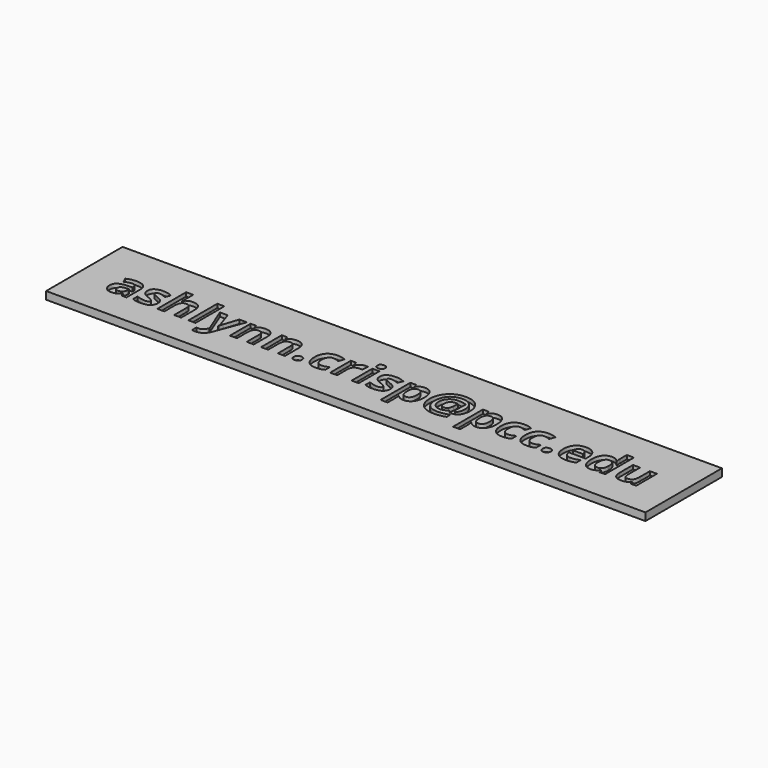
from build123d import *

# Parameters (mm, degrees)
F0_W         = 78
F0_H         = 12.4420574262
F0_W_2       = 0.9186807134
F0_H_2       = 3.3681746196
F0_H_3       = 4.6878744061
F0_TEXT_SIZE = 6.169524203
F1_DEPTH     = 1
F2_DEPTH     = 0.5


# Not quite as in the source:
# - Text() gives the source's letters only with a copy of the font that has no kerning and outlines rounded to 1/6400 em; it was checked with that copy


with BuildPart() as f1:
    # F0 (on Top) → F1 (new body)
    with BuildSketch(Plane.XY):
        with Locations((0, 2.2210287131)):
            Rectangle(F0_W, F0_H)
        with BuildLine():
            Line((-31.7378640777, 0), (-32.3789162019, 0))
            Line((-32.3789162019, 0), (-32.5572540109, 0.4578943744))
            Line((-32.5572540109, 0.4578943744), (-32.5813537148, 0.4578943744))
            add(Edge.make_bspline(
                [(-32.5813537148, 0.4578943744), (-32.8127108724, 0.165805963), (-33.0585278524, 0.0525373545)],
                knots=[0, 0, 0, 1, 1, 1], degree=2))
            add(Edge.make_bspline(
                [(-33.0585278524, 0.0525373545), (-33.3043448323, -0.0607312539), (-33.6986159884, -0.0607312539)],
                knots=[0, 0, 0, 1, 1, 1], degree=2))
            add(Edge.make_bspline(
                [(-33.6986159884, -0.0607312539), (-34.1835020313, -0.0607312539), (-34.4620946086, 0.2168973353)],
                knots=[0, 0, 0, 1, 1, 1], degree=2))
            add(Edge.make_bspline(
                [(-34.4620946086, 0.2168973353), (-34.7406871858, 0.4945259244), (-34.7406871858, 1.0064036356)],
                knots=[0, 0, 0, 1, 1, 1], degree=2))
            add(Edge.make_bspline(
                [(-34.7406871858, 1.0064036356), (-34.7406871858, 1.5423810507), (-34.3656957929, 1.7968739241)],
                knots=[0, 0, 0, 1, 1, 1], degree=2))
            add(Edge.make_bspline(
                [(-34.3656957929, 1.7968739241), (-33.9907043999, 2.0513667975), (-33.2349376851, 2.0783584659)],
                knots=[0, 0, 0, 1, 1, 1], degree=2))
            Line((-33.2349376851, 2.0783584659), (-32.6497968739, 2.0966742409))
            Line((-32.6497968739, 2.0966742409), (-32.6497968739, 2.2441644288))
            add(Edge.make_bspline(
                [(-32.6497968739, 2.2441644288), (-32.6497968739, 2.7560421401), (-33.1742064312, 2.7560421401)],
                knots=[0, 0, 0, 1, 1, 1], degree=2))
            add(Edge.make_bspline(
                [(-33.1742064312, 2.7560421401), (-33.5781174688, 2.7560421401), (-34.1237347655, 2.5121531364)],
                knots=[0, 0, 0, 1, 1, 1], degree=2))
            Line((-34.1237347655, 2.5121531364), (-34.4273910349, 3.1329615093))
            add(Edge.make_bspline(
                [(-34.4273910349, 3.1329615093), (-33.8461061764, 3.4375817669), (-33.1385388694, 3.4375817669)],
                knots=[0, 0, 0, 1, 1, 1], degree=2))
            add(Edge.make_bspline(
                [(-33.1385388694, 3.4375817669), (-32.4608551952, 3.4375817669), (-32.0993596364, 3.1421193968)],
                knots=[0, 0, 0, 1, 1, 1], degree=2))
            add(Edge.make_bspline(
                [(-32.0993596364, 3.1421193968), (-31.7378640777, 2.8466570268), (-31.7378640777, 2.2441644288)],
                knots=[0, 0, 0, 1, 1, 1], degree=2))
            Line((-31.7378640777, 2.2441644288), (-31.7378640777, 0))
        make_face(mode=Mode.SUBTRACT)
        with BuildLine():
            add(Edge.make_bspline(
                [(-28.528747504, 1.4310404186), (-28.4410245817, 1.2502926393), (-28.4410245817, 1.0006197067)],
                knots=[0, 0, 0, 1, 1, 1], degree=2))
            add(Edge.make_bspline(
                [(-28.4410245817, 1.0006197067), (-28.4410245817, 0.4819940784), (-28.8010741582, 0.2106314122)],
                knots=[0, 0, 0, 1, 1, 1], degree=2))
            add(Edge.make_bspline(
                [(-28.8010741582, 0.2106314122), (-29.1611237348, -0.0607312539), (-29.8783309234, -0.0607312539)],
                knots=[0, 0, 0, 1, 1, 1], degree=2))
            add(Edge.make_bspline(
                [(-29.8783309234, -0.0607312539), (-30.2456104111, -0.0607312539), (-30.5049232252, -0.0106038697)],
                knots=[0, 0, 0, 1, 1, 1], degree=2))
            add(Edge.make_bspline(
                [(-30.5049232252, -0.0106038697), (-30.7642360394, 0.0395235144), (-30.9898092681, 0.1359223301)],
                knots=[0, 0, 0, 1, 1, 1], degree=2))
            Line((-30.9898092681, 0.1359223301), (-30.9898092681, 0.8945810094))
            add(Edge.make_bspline(
                [(-30.9898092681, 0.8945810094), (-30.7343524065, 0.7740824898), (-30.4133443503, 0.6926254906)],
                knots=[0, 0, 0, 1, 1, 1], degree=2))
            add(Edge.make_bspline(
                [(-30.4133443503, 0.6926254906), (-30.0923362942, 0.6111684914), (-29.8484472905, 0.6111684914)],
                knots=[0, 0, 0, 1, 1, 1], degree=2))
            add(Edge.make_bspline(
                [(-29.8484472905, 0.6111684914), (-29.3481374372, 0.6111684914), (-29.3481374372, 0.9003649384)],
                knots=[0, 0, 0, 1, 1, 1], degree=2))
            add(Edge.make_bspline(
                [(-29.3481374372, 0.9003649384), (-29.3481374372, 1.0092956001), (-29.41465262, 1.0772567651)],
                knots=[0, 0, 0, 1, 1, 1], degree=2))
            add(Edge.make_bspline(
                [(-29.41465262, 1.0772567651), (-29.4811678028, 1.1452179302), (-29.6435998072, 1.2310128761)],
                knots=[0, 0, 0, 1, 1, 1], degree=2))
            add(Edge.make_bspline(
                [(-29.6435998072, 1.2310128761), (-29.8060318116, 1.3168078221), (-30.0769124836, 1.4305584246)],
                knots=[0, 0, 0, 1, 1, 1], degree=2))
            add(Edge.make_bspline(
                [(-30.0769124836, 1.4305584246), (-30.4653997108, 1.5934724231), (-30.6480754665, 1.7322867176)],
                knots=[0, 0, 0, 1, 1, 1], degree=2))
            add(Edge.make_bspline(
                [(-30.6480754665, 1.7322867176), (-30.8307512222, 1.8711010122), (-30.9131722096, 2.0504028093)],
                knots=[0, 0, 0, 1, 1, 1], degree=2))
            add(Edge.make_bspline(
                [(-30.9131722096, 2.0504028093), (-30.995593197, 2.2297046065), (-30.995593197, 2.490945397)],
                knots=[0, 0, 0, 1, 1, 1], degree=2))
            add(Edge.make_bspline(
                [(-30.995593197, 2.490945397), (-30.995593197, 2.940163878), (-30.6480754665, 3.1854988639)],
                knots=[0, 0, 0, 1, 1, 1], degree=2))
            add(Edge.make_bspline(
                [(-30.6480754665, 3.1854988639), (-30.300557736, 3.4308338498), (-29.6614335881, 3.4308338498)],
                knots=[0, 0, 0, 1, 1, 1], degree=2))
            add(Edge.make_bspline(
                [(-29.6614335881, 3.4308338498), (-29.0531570612, 3.4308338498), (-28.4776561317, 3.1657371067)],
                knots=[0, 0, 0, 1, 1, 1], degree=2))
            Line((-28.4776561317, 3.1657371067), (-28.7543207326, 2.503477243))
            add(Edge.make_bspline(
                [(-28.7543207326, 2.503477243), (-29.0078496178, 2.6114439165), (-29.2276389176, 2.6808510638)],
                knots=[0, 0, 0, 1, 1, 1], degree=2))
            add(Edge.make_bspline(
                [(-29.2276389176, 2.6808510638), (-29.4474282173, 2.7502582111), (-29.6768573986, 2.7502582111)],
                knots=[0, 0, 0, 1, 1, 1], degree=2))
            add(Edge.make_bspline(
                [(-29.6768573986, 2.7502582111), (-30.0836604007, 2.7502582111), (-30.0836604007, 2.5304689114)],
                knots=[0, 0, 0, 1, 1, 1], degree=2))
            add(Edge.make_bspline(
                [(-30.0836604007, 2.5304689114), (-30.0836604007, 2.4070784273), (-29.9525580114, 2.3164635406)],
                knots=[0, 0, 0, 1, 1, 1], degree=2))
            add(Edge.make_bspline(
                [(-29.9525580114, 2.3164635406), (-29.8214556221, 2.2258486539), (-29.37802107, 2.048474833)],
                knots=[0, 0, 0, 1, 1, 1], degree=2))
            add(Edge.make_bspline(
                [(-29.37802107, 2.048474833), (-28.9837499139, 1.888452799), (-28.8001101701, 1.7501204985)],
                knots=[0, 0, 0, 1, 1, 1], degree=2))
            add(Edge.make_bspline(
                [(-28.8001101701, 1.7501204985), (-28.6164704262, 1.611788198), (-28.528747504, 1.4310404186)],
                knots=[0, 0, 0, 1, 1, 1], degree=2))
        make_face(mode=Mode.SUBTRACT)
        with BuildLine():
            Line((-20.9315568409, 0.0240997039), (-22.2695724024, 3.3681746196))
            Line((-22.2695724024, 3.3681746196), (-21.2631687668, 3.3681746196))
            Line((-21.2631687668, 3.3681746196), (-20.6279005715, 1.4729739035))
            add(Edge.make_bspline(
                [(-20.6279005715, 1.4729739035), (-20.5459615782, 1.2261929353), (-20.5160779453, 0.8887970805)],
                knots=[0, 0, 0, 1, 1, 1], degree=2))
            Line((-20.5160779453, 0.8887970805), (-20.4977621704, 0.8887970805))
            add(Edge.make_bspline(
                [(-20.4977621704, 0.8887970805), (-20.464986573, 1.199201267), (-20.3685877574, 1.4729739035)],
                knots=[0, 0, 0, 1, 1, 1], degree=2))
            Line((-20.3685877574, 1.4729739035), (-19.74488742, 3.3681746196))
            Line((-19.74488742, 3.3681746196), (-18.7596915238, 3.3681746196))
            Line((-18.7596915238, 3.3681746196), (-20.1844660194, -0.4309027061))
            add(Edge.make_bspline(
                [(-20.1844660194, -0.4309027061), (-20.3811196034, -0.9582042278), (-20.7440611444, -1.2204090064)],
                knots=[0, 0, 0, 1, 1, 1], degree=2))
            add(Edge.make_bspline(
                [(-20.7440611444, -1.2204090064), (-21.1070026854, -1.482613785), (-21.5918887282, -1.482613785)],
                knots=[0, 0, 0, 1, 1, 1], degree=2))
            add(Edge.make_bspline(
                [(-21.5918887282, -1.482613785), (-21.8299938029, -1.482613785), (-22.0584589961, -1.4305584246)],
                knots=[0, 0, 0, 1, 1, 1], degree=2))
            Line((-22.0584589961, -1.4305584246), (-22.0584589961, -0.7017833781))
            add(Edge.make_bspline(
                [(-22.0584589961, -0.7017833781), (-21.8926530331, -0.7413068925), (-21.6969634373, -0.7413068925)],
                knots=[0, 0, 0, 1, 1, 1], degree=2))
            add(Edge.make_bspline(
                [(-21.6969634373, -0.7413068925), (-21.4530744337, -0.7413068925), (-21.270880672, -0.5918887282)],
                knots=[0, 0, 0, 1, 1, 1], degree=2))
            add(Edge.make_bspline(
                [(-21.270880672, -0.5918887282), (-21.0886869104, -0.4424705639), (-20.9865041658, -0.141706259)],
                knots=[0, 0, 0, 1, 1, 1], degree=2))
            Line((-20.9865041658, -0.141706259), (-20.9315568409, 0.0240997039))
        make_face(mode=Mode.SUBTRACT)
        with BuildLine():
            add(Edge.make_bspline(
                [(-10.1594711836, 0.0530193486), (-10.2978034841, 0.1870137024), (-10.2978034841, 0.4309027061)],
                knots=[0, 0, 0, 1, 1, 1], degree=2))
            add(Edge.make_bspline(
                [(-10.2978034841, 0.4309027061), (-10.2978034841, 0.6834676031), (-10.1623631481, 0.8131240102)],
                knots=[0, 0, 0, 1, 1, 1], degree=2))
            add(Edge.make_bspline(
                [(-10.1623631481, 0.8131240102), (-10.0269228121, 0.9427804173), (-9.7676099979, 0.9427804173)],
                knots=[0, 0, 0, 1, 1, 1], degree=2))
            add(Edge.make_bspline(
                [(-9.7676099979, 0.9427804173), (-9.5179370653, 0.9427804173), (-9.3810507471, 0.8102320457)],
                knots=[0, 0, 0, 1, 1, 1], degree=2))
            add(Edge.make_bspline(
                [(-9.3810507471, 0.8102320457), (-9.2441644288, 0.6776836742), (-9.2441644288, 0.4309027061)],
                knots=[0, 0, 0, 1, 1, 1], degree=2))
            add(Edge.make_bspline(
                [(-9.2441644288, 0.4309027061), (-9.2441644288, 0.1927976313), (-9.3824967293, 0.0559113131)],
                knots=[0, 0, 0, 1, 1, 1], degree=2))
            add(Edge.make_bspline(
                [(-9.3824967293, 0.0559113131), (-9.5208290298, -0.0809750052), (-9.7676099979, -0.0809750052)],
                knots=[0, 0, 0, 1, 1, 1], degree=2))
            add(Edge.make_bspline(
                [(-9.7676099979, -0.0809750052), (-10.0211388832, -0.0809750052), (-10.1594711836, 0.0530193486)],
                knots=[0, 0, 0, 1, 1, 1], degree=2))
        make_face(mode=Mode.SUBTRACT)
        with BuildLine():
            Line((-15.16883564, 2.195965021), (-15.16883564, 0))
            Line((-15.16883564, 0), (-16.0875163534, 0))
            Line((-16.0875163534, 0), (-16.0875163534, 1.9674998279))
            add(Edge.make_bspline(
                [(-16.0875163534, 1.9674998279), (-16.0875163534, 2.3318873511), (-16.2171727604, 2.5140811127)],
                knots=[0, 0, 0, 1, 1, 1], degree=2))
            add(Edge.make_bspline(
                [(-16.2171727604, 2.5140811127), (-16.3468291675, 2.6962748743), (-16.6302416856, 2.6962748743)],
                knots=[0, 0, 0, 1, 1, 1], degree=2))
            add(Edge.make_bspline(
                [(-16.6302416856, 2.6962748743), (-17.0158369483, 2.6962748743), (-17.1874268402, 2.4388900365)],
                knots=[0, 0, 0, 1, 1, 1], degree=2))
            add(Edge.make_bspline(
                [(-17.1874268402, 2.4388900365), (-17.3590167321, 2.1815051987), (-17.3590167321, 1.5847965296)],
                knots=[0, 0, 0, 1, 1, 1], degree=2))
            Line((-17.3590167321, 1.5847965296), (-17.3590167321, 0))
            Line((-17.3590167321, 0), (-18.2776974454, 0))
            Line((-18.2776974454, 0), (-18.2776974454, 3.3681746196))
            Line((-18.2776974454, 3.3681746196), (-17.5759140673, 3.3681746196))
            Line((-17.5759140673, 3.3681746196), (-17.4525235833, 2.9372719135))
            Line((-17.4525235833, 2.9372719135), (-17.401432211, 2.9372719135))
            add(Edge.make_bspline(
                [(-17.401432211, 2.9372719135), (-17.2471941059, 3.1811609172), (-16.9777594161, 3.3059973835)],
                knots=[0, 0, 0, 1, 1, 1], degree=2))
            add(Edge.make_bspline(
                [(-16.9777594161, 3.3059973835), (-16.7083247263, 3.4308338498), (-16.3651449425, 3.4308338498)],
                knots=[0, 0, 0, 1, 1, 1], degree=2))
            add(Edge.make_bspline(
                [(-16.3651449425, 3.4308338498), (-15.7771121669, 3.4308338498), (-15.4729739035, 3.1131997521)],
                knots=[0, 0, 0, 1, 1, 1], degree=2))
            add(Edge.make_bspline(
                [(-15.4729739035, 3.1131997521), (-15.16883564, 2.7955656545), (-15.16883564, 2.195965021)],
                knots=[0, 0, 0, 1, 1, 1], degree=2))
        make_face(mode=Mode.SUBTRACT)
        with BuildLine():
            Line((-11.1143014529, 2.195965021), (-11.1143014529, 0))
            Line((-11.1143014529, 0), (-12.0329821662, 0))
            Line((-12.0329821662, 0), (-12.0329821662, 1.9674998279))
            add(Edge.make_bspline(
                [(-12.0329821662, 1.9674998279), (-12.0329821662, 2.3318873511), (-12.1626385733, 2.5140811127)],
                knots=[0, 0, 0, 1, 1, 1], degree=2))
            add(Edge.make_bspline(
                [(-12.1626385733, 2.5140811127), (-12.2922949804, 2.6962748743), (-12.5757074985, 2.6962748743)],
                knots=[0, 0, 0, 1, 1, 1], degree=2))
            add(Edge.make_bspline(
                [(-12.5757074985, 2.6962748743), (-12.9613027611, 2.6962748743), (-13.132892653, 2.4388900365)],
                knots=[0, 0, 0, 1, 1, 1], degree=2))
            add(Edge.make_bspline(
                [(-13.132892653, 2.4388900365), (-13.3044825449, 2.1815051987), (-13.3044825449, 1.5847965296)],
                knots=[0, 0, 0, 1, 1, 1], degree=2))
            Line((-13.3044825449, 1.5847965296), (-13.3044825449, 0))
            Line((-13.3044825449, 0), (-14.2231632583, 0))
            Line((-14.2231632583, 0), (-14.2231632583, 3.3681746196))
            Line((-14.2231632583, 3.3681746196), (-13.5213798802, 3.3681746196))
            Line((-13.5213798802, 3.3681746196), (-13.3979893961, 2.9372719135))
            Line((-13.3979893961, 2.9372719135), (-13.3468980238, 2.9372719135))
            add(Edge.make_bspline(
                [(-13.3468980238, 2.9372719135), (-13.1926599187, 3.1811609172), (-12.9232252289, 3.3059973835)],
                knots=[0, 0, 0, 1, 1, 1], degree=2))
            add(Edge.make_bspline(
                [(-12.9232252289, 3.3059973835), (-12.6537905391, 3.4308338498), (-12.3106107554, 3.4308338498)],
                knots=[0, 0, 0, 1, 1, 1], degree=2))
            add(Edge.make_bspline(
                [(-12.3106107554, 3.4308338498), (-11.7225779798, 3.4308338498), (-11.4184397163, 3.1131997521)],
                knots=[0, 0, 0, 1, 1, 1], degree=2))
            add(Edge.make_bspline(
                [(-11.4184397163, 3.1131997521), (-11.1143014529, 2.7955656545), (-11.1143014529, 2.195965021)],
                knots=[0, 0, 0, 1, 1, 1], degree=2))
        make_face(mode=Mode.SUBTRACT)
        with BuildLine():
            add(Edge.make_bspline(
                [(-6.4678785375, -0.006265923), (-6.6953797425, -0.0607312539), (-7.0414514907, -0.0607312539)],
                knots=[0, 0, 0, 1, 1, 1], degree=2))
            add(Edge.make_bspline(
                [(-7.0414514907, -0.0607312539), (-8.6137161743, -0.0607312539), (-8.6137161743, 1.6657715348)],
                knots=[0, 0, 0, 1, 1, 1], degree=2))
            add(Edge.make_bspline(
                [(-8.6137161743, 1.6657715348), (-8.6137161743, 2.5246849824), (-8.1861874268, 2.9777594161)],
                knots=[0, 0, 0, 1, 1, 1], degree=2))
            add(Edge.make_bspline(
                [(-8.1861874268, 2.9777594161), (-7.7586586793, 3.4308338498), (-6.9604764856, 3.4308338498)],
                knots=[0, 0, 0, 1, 1, 1], degree=2))
            add(Edge.make_bspline(
                [(-6.9604764856, 3.4308338498), (-6.3762996626, 3.4308338498), (-5.9116573711, 3.2023686566)],
                knots=[0, 0, 0, 1, 1, 1], degree=2))
            Line((-5.9116573711, 3.2023686566), (-6.1835020313, 2.490945397))
            add(Edge.make_bspline(
                [(-6.1835020313, 2.490945397), (-6.4003993665, 2.5786683192), (-6.5869310748, 2.6345796323)],
                knots=[0, 0, 0, 1, 1, 1], degree=2))
            add(Edge.make_bspline(
                [(-6.5869310748, 2.6345796323), (-6.7734627832, 2.6904909454), (-6.9604764856, 2.6904909454)],
                knots=[0, 0, 0, 1, 1, 1], degree=2))
            add(Edge.make_bspline(
                [(-6.9604764856, 2.6904909454), (-7.6776836742, 2.6904909454), (-7.6776836742, 1.6715554637)],
                knots=[0, 0, 0, 1, 1, 1], degree=2))
            add(Edge.make_bspline(
                [(-7.6776836742, 1.6715554637), (-7.6776836742, 0.6834676031), (-6.9604764856, 0.6834676031)],
                knots=[0, 0, 0, 1, 1, 1], degree=2))
            add(Edge.make_bspline(
                [(-6.9604764856, 0.6834676031), (-6.6953797425, 0.6834676031), (-6.4693245197, 0.7543207326)],
                knots=[0, 0, 0, 1, 1, 1], degree=2))
            add(Edge.make_bspline(
                [(-6.4693245197, 0.7543207326), (-6.243269297, 0.8251738621), (-6.0176960683, 0.9765200028)],
                knots=[0, 0, 0, 1, 1, 1], degree=2))
            Line((-6.0176960683, 0.9765200028), (-6.0176960683, 0.1899056669))
            add(Edge.make_bspline(
                [(-6.0176960683, 0.1899056669), (-6.2403773325, 0.0481994078), (-6.4678785375, -0.006265923)],
                knots=[0, 0, 0, 1, 1, 1], degree=2))
        make_face(mode=Mode.SUBTRACT)
        with BuildLine():
            add(Edge.make_bspline(
                [(-3.936927632, 3.2577979756), (-3.6703849067, 3.4308338498), (-3.3570887558, 3.4308338498)],
                knots=[0, 0, 0, 1, 1, 1], degree=2))
            add(Edge.make_bspline(
                [(-3.3570887558, 3.4308338498), (-3.1700750534, 3.4308338498), (-3.0466845693, 3.4038421814)],
                knots=[0, 0, 0, 1, 1, 1], degree=2))
            Line((-3.0466845693, 3.4038421814), (-3.1160917166, 2.5430007574))
            add(Edge.make_bspline(
                [(-3.1160917166, 2.5430007574), (-3.2279143428, 2.5728843903), (-3.3869723886, 2.5728843903)],
                knots=[0, 0, 0, 1, 1, 1], degree=2))
            add(Edge.make_bspline(
                [(-3.3869723886, 2.5728843903), (-3.8265509881, 2.5728843903), (-4.0723679681, 2.3468291675)],
                knots=[0, 0, 0, 1, 1, 1], degree=2))
            add(Edge.make_bspline(
                [(-4.0723679681, 2.3468291675), (-4.318184948, 2.1207739448), (-4.318184948, 1.7139709426)],
                knots=[0, 0, 0, 1, 1, 1], degree=2))
            Line((-4.318184948, 1.7139709426), (-4.318184948, 0))
            Line((-4.318184948, 0), (-5.2368656614, 0))
            Line((-5.2368656614, 0), (-5.2368656614, 3.3681746196))
            Line((-5.2368656614, 3.3681746196), (-4.5408662122, 3.3681746196))
            Line((-4.5408662122, 3.3681746196), (-4.4049438821, 2.8013495834))
            Line((-4.4049438821, 2.8013495834), (-4.3606004269, 2.8013495834))
            add(Edge.make_bspline(
                [(-4.3606004269, 2.8013495834), (-4.2034703574, 3.0847621015), (-3.936927632, 3.2577979756)],
                knots=[0, 0, 0, 1, 1, 1], degree=2))
        make_face(mode=Mode.SUBTRACT)
        with Locations((-1.9761757213, 1.6840873098)):
            Rectangle(F0_W_2, F0_H_2, mode=Mode.SUBTRACT)
        with BuildLine():
            add(Edge.make_bspline(
                [(5.049851959, 0.147490188), (4.7577635475, -0.0607312539), (4.3634923914, -0.0607312539)],
                knots=[0, 0, 0, 1, 1, 1], degree=2))
            add(Edge.make_bspline(
                [(4.3634923914, -0.0607312539), (3.7696756868, -0.0607312539), (3.432279832, 0.3701714522)],
                knots=[0, 0, 0, 1, 1, 1], degree=2))
            Line((3.432279832, 0.3701714522), (3.3840804242, 0.3701714522))
            add(Edge.make_bspline(
                [(3.3840804242, 0.3701714522), (3.432279832, -0.0510913723), (3.432279832, -0.1176065551)],
                knots=[0, 0, 0, 1, 1, 1], degree=2))
            Line((3.432279832, -0.1176065551), (3.432279832, -1.482613785))
            Line((3.432279832, -1.482613785), (2.5135991186, -1.482613785))
            Line((2.5135991186, -1.482613785), (2.5135991186, 3.3681746196))
            Line((2.5135991186, 3.3681746196), (3.2606899401, 3.3681746196))
            Line((3.2606899401, 3.3681746196), (3.3898643531, 2.9314879846))
            Line((3.3898643531, 2.9314879846), (3.432279832, 2.9314879846))
            add(Edge.make_bspline(
                [(3.432279832, 2.9314879846), (3.7552158645, 3.4308338498), (4.3875920953, 3.4308338498)],
                knots=[0, 0, 0, 1, 1, 1], degree=2))
            add(Edge.make_bspline(
                [(4.3875920953, 3.4308338498), (4.9843007643, 3.4308338498), (5.3216966192, 2.9700475108)],
                knots=[0, 0, 0, 1, 1, 1], degree=2))
            add(Edge.make_bspline(
                [(5.3216966192, 2.9700475108), (5.659092474, 2.5092611719), (5.659092474, 1.6898712387)],
                knots=[0, 0, 0, 1, 1, 1], degree=2))
            add(Edge.make_bspline(
                [(5.659092474, 1.6898712387), (5.659092474, 1.1510018591), (5.5005164222, 0.7533567445)],
                knots=[0, 0, 0, 1, 1, 1], degree=2))
            add(Edge.make_bspline(
                [(5.5005164222, 0.7533567445), (5.3419403704, 0.3557116298), (5.049851959, 0.147490188)],
                knots=[0, 0, 0, 1, 1, 1], degree=2))
        make_face(mode=Mode.SUBTRACT)
        with BuildLine():
            add(Edge.make_bspline(
                [(1.7096329959, 1.4310404186), (1.7973559182, 1.2502926393), (1.7973559182, 1.0006197067)],
                knots=[0, 0, 0, 1, 1, 1], degree=2))
            add(Edge.make_bspline(
                [(1.7973559182, 1.0006197067), (1.7973559182, 0.4819940784), (1.4373063417, 0.2106314122)],
                knots=[0, 0, 0, 1, 1, 1], degree=2))
            add(Edge.make_bspline(
                [(1.4373063417, 0.2106314122), (1.0772567651, -0.0607312539), (0.3600495765, -0.0607312539)],
                knots=[0, 0, 0, 1, 1, 1], degree=2))
            add(Edge.make_bspline(
                [(0.3600495765, -0.0607312539), (-0.0072299112, -0.0607312539), (-0.2665427253, -0.0106038697)],
                knots=[0, 0, 0, 1, 1, 1], degree=2))
            add(Edge.make_bspline(
                [(-0.2665427253, -0.0106038697), (-0.5258555395, 0.0395235144), (-0.7514287682, 0.1359223301)],
                knots=[0, 0, 0, 1, 1, 1], degree=2))
            Line((-0.7514287682, 0.1359223301), (-0.7514287682, 0.8945810094))
            add(Edge.make_bspline(
                [(-0.7514287682, 0.8945810094), (-0.4959719066, 0.7740824898), (-0.1749638504, 0.6926254906)],
                knots=[0, 0, 0, 1, 1, 1], degree=2))
            add(Edge.make_bspline(
                [(-0.1749638504, 0.6926254906), (0.1460442057, 0.6111684914), (0.3899332094, 0.6111684914)],
                knots=[0, 0, 0, 1, 1, 1], degree=2))
            add(Edge.make_bspline(
                [(0.3899332094, 0.6111684914), (0.8902430627, 0.6111684914), (0.8902430627, 0.9003649384)],
                knots=[0, 0, 0, 1, 1, 1], degree=2))
            add(Edge.make_bspline(
                [(0.8902430627, 0.9003649384), (0.8902430627, 1.0092956001), (0.8237278799, 1.0772567651)],
                knots=[0, 0, 0, 1, 1, 1], degree=2))
            add(Edge.make_bspline(
                [(0.8237278799, 1.0772567651), (0.7572126971, 1.1452179302), (0.5947806927, 1.2310128761)],
                knots=[0, 0, 0, 1, 1, 1], degree=2))
            add(Edge.make_bspline(
                [(0.5947806927, 1.2310128761), (0.4323486883, 1.3168078221), (0.1614680163, 1.4305584246)],
                knots=[0, 0, 0, 1, 1, 1], degree=2))
            add(Edge.make_bspline(
                [(0.1614680163, 1.4305584246), (-0.2270192109, 1.5934724231), (-0.4096949666, 1.7322867176)],
                knots=[0, 0, 0, 1, 1, 1], degree=2))
            add(Edge.make_bspline(
                [(-0.4096949666, 1.7322867176), (-0.5923707223, 1.8711010122), (-0.6747917097, 2.0504028093)],
                knots=[0, 0, 0, 1, 1, 1], degree=2))
            add(Edge.make_bspline(
                [(-0.6747917097, 2.0504028093), (-0.7572126971, 2.2297046065), (-0.7572126971, 2.490945397)],
                knots=[0, 0, 0, 1, 1, 1], degree=2))
            add(Edge.make_bspline(
                [(-0.7572126971, 2.490945397), (-0.7572126971, 2.940163878), (-0.4096949666, 3.1854988639)],
                knots=[0, 0, 0, 1, 1, 1], degree=2))
            add(Edge.make_bspline(
                [(-0.4096949666, 3.1854988639), (-0.0621772361, 3.4308338498), (0.5769469118, 3.4308338498)],
                knots=[0, 0, 0, 1, 1, 1], degree=2))
            add(Edge.make_bspline(
                [(0.5769469118, 3.4308338498), (1.1852234387, 3.4308338498), (1.7607243682, 3.1657371067)],
                knots=[0, 0, 0, 1, 1, 1], degree=2))
            Line((1.7607243682, 3.1657371067), (1.4840597673, 2.503477243))
            add(Edge.make_bspline(
                [(1.4840597673, 2.503477243), (1.230530882, 2.6114439165), (1.0107415823, 2.6808510638)],
                knots=[0, 0, 0, 1, 1, 1], degree=2))
            add(Edge.make_bspline(
                [(1.0107415823, 2.6808510638), (0.7909522826, 2.7502582111), (0.5615231013, 2.7502582111)],
                knots=[0, 0, 0, 1, 1, 1], degree=2))
            add(Edge.make_bspline(
                [(0.5615231013, 2.7502582111), (0.1547200992, 2.7502582111), (0.1547200992, 2.5304689114)],
                knots=[0, 0, 0, 1, 1, 1], degree=2))
            add(Edge.make_bspline(
                [(0.1547200992, 2.5304689114), (0.1547200992, 2.4070784273), (0.2858224885, 2.3164635406)],
                knots=[0, 0, 0, 1, 1, 1], degree=2))
            add(Edge.make_bspline(
                [(0.2858224885, 2.3164635406), (0.4169248778, 2.2258486539), (0.8603594299, 2.048474833)],
                knots=[0, 0, 0, 1, 1, 1], degree=2))
            add(Edge.make_bspline(
                [(0.8603594299, 2.048474833), (1.254630586, 1.888452799), (1.4382703298, 1.7501204985)],
                knots=[0, 0, 0, 1, 1, 1], degree=2))
            add(Edge.make_bspline(
                [(1.4382703298, 1.7501204985), (1.6219100737, 1.611788198), (1.7096329959, 1.4310404186)],
                knots=[0, 0, 0, 1, 1, 1], degree=2))
        make_face(mode=Mode.SUBTRACT)
        with BuildLine():
            add(Edge.make_bspline(
                [(10.8790883426, 3.4192659919), (11.1625008607, 2.9189561385), (11.1625008607, 2.2653721683)],
                knots=[0, 0, 0, 1, 1, 1], degree=2))
            add(Edge.make_bspline(
                [(11.1625008607, 2.2653721683), (11.1625008607, 1.8315774978), (11.0236865661, 1.4715279212)],
                knots=[0, 0, 0, 1, 1, 1], degree=2))
            add(Edge.make_bspline(
                [(11.0236865661, 1.4715279212), (10.8848722716, 1.1114783447), (10.6318253804, 0.9066308614)],
                knots=[0, 0, 0, 1, 1, 1], degree=2))
            add(Edge.make_bspline(
                [(10.6318253804, 0.9066308614), (10.3787784893, 0.7017833781), (10.0452385871, 0.7017833781)],
                knots=[0, 0, 0, 1, 1, 1], degree=2))
            add(Edge.make_bspline(
                [(10.0452385871, 0.7017833781), (9.8215933347, 0.7017833781), (9.6500034428, 0.8087860635)],
                knots=[0, 0, 0, 1, 1, 1], degree=2))
            add(Edge.make_bspline(
                [(9.6500034428, 0.8087860635), (9.4784135509, 0.9157887489), (9.4032224747, 1.0902706052)],
                knots=[0, 0, 0, 1, 1, 1], degree=2))
            Line((9.4032224747, 1.0902706052), (9.3550230669, 1.0902706052))
            add(Edge.make_bspline(
                [(9.3550230669, 1.0902706052), (9.0291950699, 0.7017833781), (8.5269572402, 0.7017833781)],
                knots=[0, 0, 0, 1, 1, 1], degree=2))
            add(Edge.make_bspline(
                [(8.5269572402, 0.7017833781), (7.9929078014, 0.7017833781), (7.6858775735, 1.0227914343)],
                knots=[0, 0, 0, 1, 1, 1], degree=2))
            add(Edge.make_bspline(
                [(7.6858775735, 1.0227914343), (7.3788473456, 1.3437994905), (7.3788473456, 1.900984645)],
                knots=[0, 0, 0, 1, 1, 1], degree=2))
            add(Edge.make_bspline(
                [(7.3788473456, 1.900984645), (7.3788473456, 2.5362528403), (7.7822763892, 2.9252220616)],
                knots=[0, 0, 0, 1, 1, 1], degree=2))
            add(Edge.make_bspline(
                [(7.7822763892, 2.9252220616), (8.1857054328, 3.3141912828), (8.8363974385, 3.3141912828)],
                knots=[0, 0, 0, 1, 1, 1], degree=2))
            add(Edge.make_bspline(
                [(8.8363974385, 3.3141912828), (9.0957102527, 3.3141912828), (9.4075604214, 3.2640638986)],
                knots=[0, 0, 0, 1, 1, 1], degree=2))
            add(Edge.make_bspline(
                [(9.4075604214, 3.2640638986), (9.7194105901, 3.2139365145), (9.9208841149, 3.1454933554)],
                knots=[0, 0, 0, 1, 1, 1], degree=2))
            Line((9.9208841149, 3.1454933554), (9.8524409557, 1.6715554637))
            add(Edge.make_bspline(
                [(9.8524409557, 1.6715554637), (9.8524409557, 1.2531846037), (10.0809061489, 1.2531846037)],
                knots=[0, 0, 0, 1, 1, 1], degree=2))
            add(Edge.make_bspline(
                [(10.0809061489, 1.2531846037), (10.2737037802, 1.2531846037), (10.3884183709, 1.5346691455)],
                knots=[0, 0, 0, 1, 1, 1], degree=2))
            add(Edge.make_bspline(
                [(10.3884183709, 1.5346691455), (10.5031329615, 1.8161536873), (10.5031329615, 2.2711560972)],
                knots=[0, 0, 0, 1, 1, 1], degree=2))
            add(Edge.make_bspline(
                [(10.5031329615, 2.2711560972), (10.5031329615, 2.7560421401), (10.3011774427, 3.1281415685)],
                knots=[0, 0, 0, 1, 1, 1], degree=2))
            add(Edge.make_bspline(
                [(10.3011774427, 3.1281415685), (10.0992219238, 3.500240997), (9.7329064243, 3.6964125869)],
                knots=[0, 0, 0, 1, 1, 1], degree=2))
            add(Edge.make_bspline(
                [(9.7329064243, 3.6964125869), (9.3665909247, 3.8925841768), (8.8971286924, 3.8925841768)],
                knots=[0, 0, 0, 1, 1, 1], degree=2))
            add(Edge.make_bspline(
                [(8.8971286924, 3.8925841768), (8.2888521655, 3.8925841768), (7.8396336845, 3.6424292502)],
                knots=[0, 0, 0, 1, 1, 1], degree=2))
            add(Edge.make_bspline(
                [(7.8396336845, 3.6424292502), (7.3904152035, 3.3922743235), (7.1513461406, 2.9208841149)],
                knots=[0, 0, 0, 1, 1, 1], degree=2))
            add(Edge.make_bspline(
                [(7.1513461406, 2.9208841149), (6.9122770777, 2.4494939062), (6.9122770777, 1.8315774978)],
                knots=[0, 0, 0, 1, 1, 1], degree=2))
            add(Edge.make_bspline(
                [(6.9122770777, 1.8315774978), (6.9122770777, 1.0006197067), (7.3561936239, 0.5562211664)],
                knots=[0, 0, 0, 1, 1, 1], degree=2))
            add(Edge.make_bspline(
                [(7.3561936239, 0.5562211664), (7.8001101701, 0.1118226262), (8.6435998072, 0.1118226262)],
                knots=[0, 0, 0, 1, 1, 1], degree=2))
            add(Edge.make_bspline(
                [(8.6435998072, 0.1118226262), (8.9636438752, 0.1118226262), (9.3458651794, 0.1826757557)],
                knots=[0, 0, 0, 1, 1, 1], degree=2))
            add(Edge.make_bspline(
                [(9.3458651794, 0.1826757557), (9.7280864835, 0.2535288852), (10.0992219238, 0.3884872272)],
                knots=[0, 0, 0, 1, 1, 1], degree=2))
            Line((10.0992219238, 0.3884872272), (10.0992219238, -0.1899056669))
            add(Edge.make_bspline(
                [(10.0992219238, -0.1899056669), (9.454313847, -0.4636783034), (8.6676995111, -0.4636783034)],
                knots=[0, 0, 0, 1, 1, 1], degree=2))
            add(Edge.make_bspline(
                [(8.6676995111, -0.4636783034), (7.5234455691, -0.4636783034), (6.883357433, 0.1388142946)],
                knots=[0, 0, 0, 1, 1, 1], degree=2))
            add(Edge.make_bspline(
                [(6.883357433, 0.1388142946), (6.243269297, 0.7413068925), (6.243269297, 1.8132617228)],
                knots=[0, 0, 0, 1, 1, 1], degree=2))
            add(Edge.make_bspline(
                [(6.243269297, 1.8132617228), (6.243269297, 2.5574605798), (6.5700612821, 3.1647731185)],
                knots=[0, 0, 0, 1, 1, 1], degree=2))
            add(Edge.make_bspline(
                [(6.5700612821, 3.1647731185), (6.8968532672, 3.7720856572), (7.5007918474, 4.1167114233)],
                knots=[0, 0, 0, 1, 1, 1], degree=2))
            add(Edge.make_bspline(
                [(7.5007918474, 4.1167114233), (8.1047304276, 4.4613371893), (8.8913447635, 4.4613371893)],
                knots=[0, 0, 0, 1, 1, 1], degree=2))
            add(Edge.make_bspline(
                [(8.8913447635, 4.4613371893), (9.5536046271, 4.4613371893), (10.0746402258, 4.1904565172)],
                knots=[0, 0, 0, 1, 1, 1], degree=2))
            add(Edge.make_bspline(
                [(10.0746402258, 4.1904565172), (10.5956758246, 3.9195758452), (10.8790883426, 3.4192659919)],
                knots=[0, 0, 0, 1, 1, 1], degree=2))
        make_face(mode=Mode.SUBTRACT)
        with BuildLine():
            add(Edge.make_bspline(
                [(14.4882600014, 0.147490188), (14.1961715899, -0.0607312539), (13.8019004338, -0.0607312539)],
                knots=[0, 0, 0, 1, 1, 1], degree=2))
            add(Edge.make_bspline(
                [(13.8019004338, -0.0607312539), (13.2080837293, -0.0607312539), (12.8706878744, 0.3701714522)],
                knots=[0, 0, 0, 1, 1, 1], degree=2))
            Line((12.8706878744, 0.3701714522), (12.8224884666, 0.3701714522))
            add(Edge.make_bspline(
                [(12.8224884666, 0.3701714522), (12.8706878744, -0.0510913723), (12.8706878744, -0.1176065551)],
                knots=[0, 0, 0, 1, 1, 1], degree=2))
            Line((12.8706878744, -0.1176065551), (12.8706878744, -1.482613785))
            Line((12.8706878744, -1.482613785), (11.9520071611, -1.482613785))
            Line((11.9520071611, -1.482613785), (11.9520071611, 3.3681746196))
            Line((11.9520071611, 3.3681746196), (12.6990979825, 3.3681746196))
            Line((12.6990979825, 3.3681746196), (12.8282723955, 2.9314879846))
            Line((12.8282723955, 2.9314879846), (12.8706878744, 2.9314879846))
            add(Edge.make_bspline(
                [(12.8706878744, 2.9314879846), (13.1936239069, 3.4308338498), (13.8260001377, 3.4308338498)],
                knots=[0, 0, 0, 1, 1, 1], degree=2))
            add(Edge.make_bspline(
                [(13.8260001377, 3.4308338498), (14.4227088067, 3.4308338498), (14.7601046616, 2.9700475108)],
                knots=[0, 0, 0, 1, 1, 1], degree=2))
            add(Edge.make_bspline(
                [(14.7601046616, 2.9700475108), (15.0975005164, 2.5092611719), (15.0975005164, 1.6898712387)],
                knots=[0, 0, 0, 1, 1, 1], degree=2))
            add(Edge.make_bspline(
                [(15.0975005164, 1.6898712387), (15.0975005164, 1.1510018591), (14.9389244646, 0.7533567445)],
                knots=[0, 0, 0, 1, 1, 1], degree=2))
            add(Edge.make_bspline(
                [(14.9389244646, 0.7533567445), (14.7803484129, 0.3557116298), (14.4882600014, 0.147490188)],
                knots=[0, 0, 0, 1, 1, 1], degree=2))
        make_face(mode=Mode.SUBTRACT)
        with BuildLine():
            add(Edge.make_bspline(
                [(17.7976313434, -0.006265923), (17.5701301384, -0.0607312539), (17.2240583901, -0.0607312539)],
                knots=[0, 0, 0, 1, 1, 1], degree=2))
            add(Edge.make_bspline(
                [(17.2240583901, -0.0607312539), (15.6517937065, -0.0607312539), (15.6517937065, 1.6657715348)],
                knots=[0, 0, 0, 1, 1, 1], degree=2))
            add(Edge.make_bspline(
                [(15.6517937065, 1.6657715348), (15.6517937065, 2.5246849824), (16.079322454, 2.9777594161)],
                knots=[0, 0, 0, 1, 1, 1], degree=2))
            add(Edge.make_bspline(
                [(16.079322454, 2.9777594161), (16.5068512015, 3.4308338498), (17.3050333953, 3.4308338498)],
                knots=[0, 0, 0, 1, 1, 1], degree=2))
            add(Edge.make_bspline(
                [(17.3050333953, 3.4308338498), (17.8892102183, 3.4308338498), (18.3538525098, 3.2023686566)],
                knots=[0, 0, 0, 1, 1, 1], degree=2))
            Line((18.3538525098, 3.2023686566), (18.0820078496, 2.490945397))
            add(Edge.make_bspline(
                [(18.0820078496, 2.490945397), (17.8651105144, 2.5786683192), (17.678578806, 2.6345796323)],
                knots=[0, 0, 0, 1, 1, 1], degree=2))
            add(Edge.make_bspline(
                [(17.678578806, 2.6345796323), (17.4920470977, 2.6904909454), (17.3050333953, 2.6904909454)],
                knots=[0, 0, 0, 1, 1, 1], degree=2))
            add(Edge.make_bspline(
                [(17.3050333953, 2.6904909454), (16.5878262067, 2.6904909454), (16.5878262067, 1.6715554637)],
                knots=[0, 0, 0, 1, 1, 1], degree=2))
            add(Edge.make_bspline(
                [(16.5878262067, 1.6715554637), (16.5878262067, 0.6834676031), (17.3050333953, 0.6834676031)],
                knots=[0, 0, 0, 1, 1, 1], degree=2))
            add(Edge.make_bspline(
                [(17.3050333953, 0.6834676031), (17.5701301384, 0.6834676031), (17.7961853612, 0.7543207326)],
                knots=[0, 0, 0, 1, 1, 1], degree=2))
            add(Edge.make_bspline(
                [(17.7961853612, 0.7543207326), (18.0222405839, 0.8251738621), (18.2478138126, 0.9765200028)],
                knots=[0, 0, 0, 1, 1, 1], degree=2))
            Line((18.2478138126, 0.9765200028), (18.2478138126, 0.1899056669))
            add(Edge.make_bspline(
                [(18.2478138126, 0.1899056669), (18.0251325484, 0.0481994078), (17.7976313434, -0.006265923)],
                knots=[0, 0, 0, 1, 1, 1], degree=2))
        make_face(mode=Mode.SUBTRACT)
        with BuildLine():
            add(Edge.make_bspline(
                [(22.2102871308, 0.0530193486), (22.0719548303, 0.1870137024), (22.0719548303, 0.4309027061)],
                knots=[0, 0, 0, 1, 1, 1], degree=2))
            add(Edge.make_bspline(
                [(22.0719548303, 0.4309027061), (22.0719548303, 0.6834676031), (22.2073951663, 0.8131240102)],
                knots=[0, 0, 0, 1, 1, 1], degree=2))
            add(Edge.make_bspline(
                [(22.2073951663, 0.8131240102), (22.3428355023, 0.9427804173), (22.6021483165, 0.9427804173)],
                knots=[0, 0, 0, 1, 1, 1], degree=2))
            add(Edge.make_bspline(
                [(22.6021483165, 0.9427804173), (22.8518212491, 0.9427804173), (22.9887075673, 0.8102320457)],
                knots=[0, 0, 0, 1, 1, 1], degree=2))
            add(Edge.make_bspline(
                [(22.9887075673, 0.8102320457), (23.1255938856, 0.6776836742), (23.1255938856, 0.4309027061)],
                knots=[0, 0, 0, 1, 1, 1], degree=2))
            add(Edge.make_bspline(
                [(23.1255938856, 0.4309027061), (23.1255938856, 0.1927976313), (22.9872615851, 0.0559113131)],
                knots=[0, 0, 0, 1, 1, 1], degree=2))
            add(Edge.make_bspline(
                [(22.9872615851, 0.0559113131), (22.8489292846, -0.0809750052), (22.6021483165, -0.0809750052)],
                knots=[0, 0, 0, 1, 1, 1], degree=2))
            add(Edge.make_bspline(
                [(22.6021483165, -0.0809750052), (22.3486194312, -0.0809750052), (22.2102871308, 0.0530193486)],
                knots=[0, 0, 0, 1, 1, 1], degree=2))
        make_face(mode=Mode.SUBTRACT)
        with BuildLine():
            add(Edge.make_bspline(
                [(20.9701163671, -0.006265923), (20.7426151622, -0.0607312539), (20.3965434139, -0.0607312539)],
                knots=[0, 0, 0, 1, 1, 1], degree=2))
            add(Edge.make_bspline(
                [(20.3965434139, -0.0607312539), (18.8242787303, -0.0607312539), (18.8242787303, 1.6657715348)],
                knots=[0, 0, 0, 1, 1, 1], degree=2))
            add(Edge.make_bspline(
                [(18.8242787303, 1.6657715348), (18.8242787303, 2.5246849824), (19.2518074778, 2.9777594161)],
                knots=[0, 0, 0, 1, 1, 1], degree=2))
            add(Edge.make_bspline(
                [(19.2518074778, 2.9777594161), (19.6793362253, 3.4308338498), (20.4775184191, 3.4308338498)],
                knots=[0, 0, 0, 1, 1, 1], degree=2))
            add(Edge.make_bspline(
                [(20.4775184191, 3.4308338498), (21.061695242, 3.4308338498), (21.5263375336, 3.2023686566)],
                knots=[0, 0, 0, 1, 1, 1], degree=2))
            Line((21.5263375336, 3.2023686566), (21.2544928734, 2.490945397))
            add(Edge.make_bspline(
                [(21.2544928734, 2.490945397), (21.0375955381, 2.5786683192), (20.8510638298, 2.6345796323)],
                knots=[0, 0, 0, 1, 1, 1], degree=2))
            add(Edge.make_bspline(
                [(20.8510638298, 2.6345796323), (20.6645321215, 2.6904909454), (20.4775184191, 2.6904909454)],
                knots=[0, 0, 0, 1, 1, 1], degree=2))
            add(Edge.make_bspline(
                [(20.4775184191, 2.6904909454), (19.7603112305, 2.6904909454), (19.7603112305, 1.6715554637)],
                knots=[0, 0, 0, 1, 1, 1], degree=2))
            add(Edge.make_bspline(
                [(19.7603112305, 1.6715554637), (19.7603112305, 0.6834676031), (20.4775184191, 0.6834676031)],
                knots=[0, 0, 0, 1, 1, 1], degree=2))
            add(Edge.make_bspline(
                [(20.4775184191, 0.6834676031), (20.7426151622, 0.6834676031), (20.9686703849, 0.7543207326)],
                knots=[0, 0, 0, 1, 1, 1], degree=2))
            add(Edge.make_bspline(
                [(20.9686703849, 0.7543207326), (21.1947256077, 0.8251738621), (21.4202988363, 0.9765200028)],
                knots=[0, 0, 0, 1, 1, 1], degree=2))
            Line((21.4202988363, 0.9765200028), (21.4202988363, 0.1899056669))
            add(Edge.make_bspline(
                [(21.4202988363, 0.1899056669), (21.1976175721, 0.0481994078), (20.9701163671, -0.006265923)],
                knots=[0, 0, 0, 1, 1, 1], degree=2))
        make_face(mode=Mode.SUBTRACT)
        with BuildLine():
            add(Edge.make_bspline(
                [(26.1534806858, -0.0019279763), (25.8797080493, -0.0607312539), (25.484472905, -0.0607312539)],
                knots=[0, 0, 0, 1, 1, 1], degree=2))
            add(Edge.make_bspline(
                [(25.484472905, -0.0607312539), (24.6718308889, -0.0607312539), (24.2139365145, 0.3884872272)],
                knots=[0, 0, 0, 1, 1, 1], degree=2))
            add(Edge.make_bspline(
                [(24.2139365145, 0.3884872272), (23.7560421401, 0.8377057082), (23.7560421401, 1.6599876059)],
                knots=[0, 0, 0, 1, 1, 1], degree=2))
            add(Edge.make_bspline(
                [(23.7560421401, 1.6599876059), (23.7560421401, 2.5063692075), (24.1792329409, 2.9686015286)],
                knots=[0, 0, 0, 1, 1, 1], degree=2))
            add(Edge.make_bspline(
                [(24.1792329409, 2.9686015286), (24.6024237417, 3.4308338498), (25.3495145631, 3.4308338498)],
                knots=[0, 0, 0, 1, 1, 1], degree=2))
            add(Edge.make_bspline(
                [(25.3495145631, 3.4308338498), (26.0628657991, 3.4308338498), (26.4605109137, 3.0245128417)],
                knots=[0, 0, 0, 1, 1, 1], degree=2))
            add(Edge.make_bspline(
                [(26.4605109137, 3.0245128417), (26.8581560284, 2.6181918336), (26.8581560284, 1.900984645)],
                knots=[0, 0, 0, 1, 1, 1], degree=2))
            Line((26.8581560284, 1.900984645), (26.8581560284, 1.4546581285))
            Line((26.8581560284, 1.4546581285), (24.6862907113, 1.4546581285))
            add(Edge.make_bspline(
                [(24.6862907113, 1.4546581285), (24.7017145218, 1.0632789369), (24.9186118571, 0.8434896371)],
                knots=[0, 0, 0, 1, 1, 1], degree=2))
            add(Edge.make_bspline(
                [(24.9186118571, 0.8434896371), (25.1355091923, 0.6237003374), (25.5268883839, 0.6237003374)],
                knots=[0, 0, 0, 1, 1, 1], degree=2))
            add(Edge.make_bspline(
                [(25.5268883839, 0.6237003374), (25.8315086415, 0.6237003374), (26.1023893135, 0.6868415617)],
                knots=[0, 0, 0, 1, 1, 1], degree=2))
            add(Edge.make_bspline(
                [(26.1023893135, 0.6868415617), (26.3732699855, 0.7499827859), (26.6682503615, 0.8887970805)],
                knots=[0, 0, 0, 1, 1, 1], degree=2))
            Line((26.6682503615, 0.8887970805), (26.6682503615, 0.1773738208))
            add(Edge.make_bspline(
                [(26.6682503615, 0.1773738208), (26.4272533223, 0.0568753012), (26.1534806858, -0.0019279763)],
                knots=[0, 0, 0, 1, 1, 1], degree=2))
        make_face(mode=Mode.SUBTRACT)
        with BuildLine():
            Line((34.599944915, 0), (33.8952695724, 0))
            Line((33.8952695724, 0), (33.7718790883, 0.4309027061))
            Line((33.7718790883, 0.4309027061), (33.7236796805, 0.4309027061))
            add(Edge.make_bspline(
                [(33.7236796805, 0.4309027061), (33.5761894925, 0.1956895958), (33.3048268264, 0.067479171)],
                knots=[0, 0, 0, 1, 1, 1], degree=2))
            add(Edge.make_bspline(
                [(33.3048268264, 0.067479171), (33.0334641603, -0.0607312539), (32.687392412, -0.0607312539)],
                knots=[0, 0, 0, 1, 1, 1], degree=2))
            add(Edge.make_bspline(
                [(32.687392412, -0.0607312539), (32.0935757075, -0.0607312539), (31.7923294085, 0.2573848378)],
                knots=[0, 0, 0, 1, 1, 1], degree=2))
            add(Edge.make_bspline(
                [(31.7923294085, 0.2573848378), (31.4910831096, 0.5755009296), (31.4910831096, 1.1722095986)],
                knots=[0, 0, 0, 1, 1, 1], degree=2))
            Line((31.4910831096, 1.1722095986), (31.4910831096, 3.3681746196))
            Line((31.4910831096, 3.3681746196), (32.4097638229, 3.3681746196))
            Line((32.4097638229, 3.3681746196), (32.4097638229, 1.4006747917))
            add(Edge.make_bspline(
                [(32.4097638229, 1.4006747917), (32.4097638229, 1.0362872685), (32.53942023, 0.8540935069)],
                knots=[0, 0, 0, 1, 1, 1], degree=2))
            add(Edge.make_bspline(
                [(32.53942023, 0.8540935069), (32.6690766371, 0.6718997452), (32.9524891551, 0.6718997452)],
                knots=[0, 0, 0, 1, 1, 1], degree=2))
            add(Edge.make_bspline(
                [(32.9524891551, 0.6718997452), (33.3380844178, 0.6718997452), (33.5096743097, 0.9292845831)],
                knots=[0, 0, 0, 1, 1, 1], degree=2))
            add(Edge.make_bspline(
                [(33.5096743097, 0.9292845831), (33.6812642016, 1.1866694209), (33.6812642016, 1.7833780899)],
                knots=[0, 0, 0, 1, 1, 1], degree=2))
            Line((33.6812642016, 1.7833780899), (33.6812642016, 3.3681746196))
            Line((33.6812642016, 3.3681746196), (34.599944915, 3.3681746196))
            Line((34.599944915, 3.3681746196), (34.599944915, 0))
        make_face(mode=Mode.SUBTRACT)
        with BuildLine():
            Line((-24.6159195758, 2.195965021), (-24.6159195758, 0))
            Line((-24.6159195758, 0), (-25.5346002892, 0))
            Line((-25.5346002892, 0), (-25.5346002892, 1.9674998279))
            add(Edge.make_bspline(
                [(-25.5346002892, 1.9674998279), (-25.5346002892, 2.6962748743), (-26.0773256214, 2.6962748743)],
                knots=[0, 0, 0, 1, 1, 1], degree=2))
            add(Edge.make_bspline(
                [(-26.0773256214, 2.6962748743), (-26.4629208841, 2.6962748743), (-26.634510776, 2.4340700957)],
                knots=[0, 0, 0, 1, 1, 1], degree=2))
            add(Edge.make_bspline(
                [(-26.634510776, 2.4340700957), (-26.8061006679, 2.1718653171), (-26.8061006679, 1.5847965296)],
                knots=[0, 0, 0, 1, 1, 1], degree=2))
            Line((-26.8061006679, 1.5847965296), (-26.8061006679, 0))
            Line((-26.8061006679, 0), (-27.7247813813, 0))
            Line((-27.7247813813, 0), (-27.7247813813, 4.6878744061))
            Line((-27.7247813813, 4.6878744061), (-26.8061006679, 4.6878744061))
            Line((-26.8061006679, 4.6878744061), (-26.8061006679, 3.7325621428))
            add(Edge.make_bspline(
                [(-26.8061006679, 3.7325621428), (-26.8061006679, 3.6207395166), (-26.8273084074, 3.2081525856)],
                knots=[0, 0, 0, 1, 1, 1], degree=2))
            Line((-26.8273084074, 3.2081525856), (-26.8485161468, 2.9372719135))
            Line((-26.8485161468, 2.9372719135), (-26.800316739, 2.9372719135))
            add(Edge.make_bspline(
                [(-26.800316739, 2.9372719135), (-26.492804517, 3.4308338498), (-25.8237967362, 3.4308338498)],
                knots=[0, 0, 0, 1, 1, 1], degree=2))
            add(Edge.make_bspline(
                [(-25.8237967362, 3.4308338498), (-25.2299800317, 3.4308338498), (-24.9229498038, 3.1117537699)],
                knots=[0, 0, 0, 1, 1, 1], degree=2))
            add(Edge.make_bspline(
                [(-24.9229498038, 3.1117537699), (-24.6159195758, 2.79267369), (-24.6159195758, 2.195965021)],
                knots=[0, 0, 0, 1, 1, 1], degree=2))
        make_face(mode=Mode.SUBTRACT)
        with Locations((-23.2109068374, 2.3439372031)):
            Rectangle(F0_W_2, F0_H_3, mode=Mode.SUBTRACT)
        with BuildLine():
            add(Edge.make_bspline(
                [(-1.974729739, 3.7865454796), (-2.4750395924, 3.7865454796), (-2.4750395924, 4.2386559251)],
                knots=[0, 0, 0, 1, 1, 1], degree=2))
            add(Edge.make_bspline(
                [(-2.4750395924, 4.2386559251), (-2.4750395924, 4.6878744061), (-1.974729739, 4.6878744061)],
                knots=[0, 0, 0, 1, 1, 1], degree=2))
            add(Edge.make_bspline(
                [(-1.974729739, 4.6878744061), (-1.4744198857, 4.6878744061), (-1.4744198857, 4.2386559251)],
                knots=[0, 0, 0, 1, 1, 1], degree=2))
            add(Edge.make_bspline(
                [(-1.4744198857, 4.2386559251), (-1.4744198857, 4.0246505543), (-1.599256352, 3.9055980169)],
                knots=[0, 0, 0, 1, 1, 1], degree=2))
            add(Edge.make_bspline(
                [(-1.599256352, 3.9055980169), (-1.7240928183, 3.7865454796), (-1.974729739, 3.7865454796)],
                knots=[0, 0, 0, 1, 1, 1], degree=2))
        make_face(mode=Mode.SUBTRACT)
        with BuildLine():
            add(Edge.make_bspline(
                [(29.6267300145, 0.436686635), (29.3134338635, -0.0607312539), (28.6714177512, -0.0607312539)],
                knots=[0, 0, 0, 1, 1, 1], degree=2))
            add(Edge.make_bspline(
                [(28.6714177512, -0.0607312539), (28.0785650348, -0.0607312539), (27.7397231977, 0.4005370791)],
                knots=[0, 0, 0, 1, 1, 1], degree=2))
            add(Edge.make_bspline(
                [(27.7397231977, 0.4005370791), (27.4008813606, 0.8618054121), (27.4008813606, 1.6783033808)],
                knots=[0, 0, 0, 1, 1, 1], degree=2))
            add(Edge.make_bspline(
                [(27.4008813606, 1.6783033808), (27.4008813606, 2.5063692075), (27.7455071266, 2.9686015286)],
                knots=[0, 0, 0, 1, 1, 1], degree=2))
            add(Edge.make_bspline(
                [(27.7455071266, 2.9686015286), (28.0901328927, 3.4308338498), (28.6955174551, 3.4308338498)],
                knots=[0, 0, 0, 1, 1, 1], degree=2))
            add(Edge.make_bspline(
                [(28.6955174551, 3.4308338498), (29.3317496385, 3.4308338498), (29.6662535289, 2.9372719135)],
                knots=[0, 0, 0, 1, 1, 1], degree=2))
            Line((29.6662535289, 2.9372719135), (29.6961371617, 2.9372719135))
            add(Edge.make_bspline(
                [(29.6961371617, 2.9372719135), (29.6267300145, 3.3141912828), (29.6267300145, 3.6091716587)],
                knots=[0, 0, 0, 1, 1, 1], degree=2))
            Line((29.6267300145, 3.6091716587), (29.6267300145, 4.6878744061))
            Line((29.6267300145, 4.6878744061), (30.5483026923, 4.6878744061))
            Line((30.5483026923, 4.6878744061), (30.5483026923, 0))
            Line((30.5483026923, 0), (29.8436273497, 0))
            Line((29.8436273497, 0), (29.6662535289, 0.436686635))
            Line((29.6662535289, 0.436686635), (29.6267300145, 0.436686635))
        make_face(mode=Mode.SUBTRACT)
        with BuildLine():
            add(Edge.make_bspline(
                [(28.5027198237, 0.9206086897), (28.6743097156, 0.6718997452), (28.9943537837, 0.6718997452)],
                knots=[0, 0, 0, 1, 1, 1], degree=2))
            add(Edge.make_bspline(
                [(28.9943537837, 0.6718997452), (29.3462094609, 0.6718997452), (29.5105694416, 0.8767472285)],
                knots=[0, 0, 0, 1, 1, 1], degree=2))
            add(Edge.make_bspline(
                [(29.5105694416, 0.8767472285), (29.6749294223, 1.0815947118), (29.6903532328, 1.5722646836)],
                knots=[0, 0, 0, 1, 1, 1], degree=2))
            Line((29.6903532328, 1.5722646836), (29.6903532328, 1.6715554637))
            add(Edge.make_bspline(
                [(29.6903532328, 1.6715554637), (29.6903532328, 2.214280796), (29.5231012876, 2.4490119121)],
                knots=[0, 0, 0, 1, 1, 1], degree=2))
            add(Edge.make_bspline(
                [(29.5231012876, 2.4490119121), (29.3558493424, 2.6837430283), (28.9789299731, 2.6837430283)],
                knots=[0, 0, 0, 1, 1, 1], degree=2))
            add(Edge.make_bspline(
                [(28.9789299731, 2.6837430283), (28.6714177512, 2.6837430283), (28.5012738415, 2.423466226)],
                knots=[0, 0, 0, 1, 1, 1], degree=2))
            add(Edge.make_bspline(
                [(28.5012738415, 2.423466226), (28.3311299318, 2.1631894237), (28.3311299318, 1.6657715348)],
                knots=[0, 0, 0, 1, 1, 1], degree=2))
            add(Edge.make_bspline(
                [(28.3311299318, 1.6657715348), (28.3311299318, 1.1693176341), (28.5027198237, 0.9206086897)],
                knots=[0, 0, 0, 1, 1, 1], degree=2))
        make_face()
        with BuildLine():
            add(Edge.make_bspline(
                [(14.0081938993, 2.4475659299), (13.8558837706, 2.6962748743), (13.5310197618, 2.6962748743)],
                knots=[0, 0, 0, 1, 1, 1], degree=2))
            add(Edge.make_bspline(
                [(13.5310197618, 2.6962748743), (13.1897679543, 2.6962748743), (13.0331198788, 2.4870894443)],
                knots=[0, 0, 0, 1, 1, 1], degree=2))
            add(Edge.make_bspline(
                [(13.0331198788, 2.4870894443), (12.8764718033, 2.2779040143), (12.8706878744, 1.795909936)],
                knots=[0, 0, 0, 1, 1, 1], degree=2))
            Line((12.8706878744, 1.795909936), (12.8706878744, 1.6956551677))
            add(Edge.make_bspline(
                [(12.8706878744, 1.6956551677), (12.8706878744, 1.1538938236), (13.0321558907, 0.9186807134)],
                knots=[0, 0, 0, 1, 1, 1], degree=2))
            add(Edge.make_bspline(
                [(13.0321558907, 0.9186807134), (13.1936239069, 0.6834676031), (13.5425876196, 0.6834676031)],
                knots=[0, 0, 0, 1, 1, 1], degree=2))
            add(Edge.make_bspline(
                [(13.5425876196, 0.6834676031), (14.1605040281, 0.6834676031), (14.1605040281, 1.7024030848)],
                knots=[0, 0, 0, 1, 1, 1], degree=2))
            add(Edge.make_bspline(
                [(14.1605040281, 1.7024030848), (14.1605040281, 2.1988569855), (14.0081938993, 2.4475659299)],
                knots=[0, 0, 0, 1, 1, 1], degree=2))
        make_face()
        with BuildLine():
            add(Edge.make_bspline(
                [(4.5697858569, 2.4475659299), (4.4174757282, 2.6962748743), (4.0926117193, 2.6962748743)],
                knots=[0, 0, 0, 1, 1, 1], degree=2))
            add(Edge.make_bspline(
                [(4.0926117193, 2.6962748743), (3.7513599119, 2.6962748743), (3.5947118364, 2.4870894443)],
                knots=[0, 0, 0, 1, 1, 1], degree=2))
            add(Edge.make_bspline(
                [(3.5947118364, 2.4870894443), (3.4380637609, 2.2779040143), (3.432279832, 1.795909936)],
                knots=[0, 0, 0, 1, 1, 1], degree=2))
            Line((3.432279832, 1.795909936), (3.432279832, 1.6956551677))
            add(Edge.make_bspline(
                [(3.432279832, 1.6956551677), (3.432279832, 1.1538938236), (3.5937478482, 0.9186807134)],
                knots=[0, 0, 0, 1, 1, 1], degree=2))
            add(Edge.make_bspline(
                [(3.5937478482, 0.9186807134), (3.7552158645, 0.6834676031), (4.1041795772, 0.6834676031)],
                knots=[0, 0, 0, 1, 1, 1], degree=2))
            add(Edge.make_bspline(
                [(4.1041795772, 0.6834676031), (4.7220959857, 0.6834676031), (4.7220959857, 1.7024030848)],
                knots=[0, 0, 0, 1, 1, 1], degree=2))
            add(Edge.make_bspline(
                [(4.7220959857, 1.7024030848), (4.7220959857, 2.1988569855), (4.5697858569, 2.4475659299)],
                knots=[0, 0, 0, 1, 1, 1], degree=2))
        make_face()
        with BuildLine():
            add(Edge.make_bspline(
                [(8.2869241892, 2.5304689114), (8.0777387592, 2.2952558011), (8.0777387592, 1.888452799)],
                knots=[0, 0, 0, 1, 1, 1], degree=2))
            add(Edge.make_bspline(
                [(8.0777387592, 1.888452799), (8.0777387592, 1.2531846037), (8.5954003994, 1.2531846037)],
                knots=[0, 0, 0, 1, 1, 1], degree=2))
            add(Edge.make_bspline(
                [(8.5954003994, 1.2531846037), (8.8672450596, 1.2531846037), (9.0084693245, 1.4445362528)],
                knots=[0, 0, 0, 1, 1, 1], degree=2))
            add(Edge.make_bspline(
                [(9.0084693245, 1.4445362528), (9.1496935895, 1.6358879019), (9.1805412105, 2.066790608)],
                knots=[0, 0, 0, 1, 1, 1], degree=2))
            Line((9.1805412105, 2.066790608), (9.2191007368, 2.7319424361))
            add(Edge.make_bspline(
                [(9.2191007368, 2.7319424361), (9.0658266198, 2.7656820216), (8.8730289885, 2.7656820216)],
                knots=[0, 0, 0, 1, 1, 1], degree=2))
            add(Edge.make_bspline(
                [(8.8730289885, 2.7656820216), (8.4961096192, 2.7656820216), (8.2869241892, 2.5304689114)],
                knots=[0, 0, 0, 1, 1, 1], degree=2))
        make_face()
        with BuildLine():
            Line((-32.6497968739, 1.2830682366), (-32.6497968739, 1.5606968257))
            Line((-32.6497968739, 1.5606968257), (-33.0055085038, 1.5481649797))
            add(Edge.make_bspline(
                [(-33.0055085038, 1.5481649797), (-33.4065275769, 1.5365971218), (-33.6022171728, 1.4040487503)],
                knots=[0, 0, 0, 1, 1, 1], degree=2))
            add(Edge.make_bspline(
                [(-33.6022171728, 1.4040487503), (-33.7979067686, 1.2715003787), (-33.7979067686, 1.0006197067)],
                knots=[0, 0, 0, 1, 1, 1], degree=2))
            add(Edge.make_bspline(
                [(-33.7979067686, 1.0006197067), (-33.7979067686, 0.6111684914), (-33.3525442402, 0.6111684914)],
                knots=[0, 0, 0, 1, 1, 1], degree=2))
            add(Edge.make_bspline(
                [(-33.3525442402, 0.6111684914), (-33.0325001721, 0.6111684914), (-32.841148523, 0.7952902293)],
                knots=[0, 0, 0, 1, 1, 1], degree=2))
            add(Edge.make_bspline(
                [(-32.841148523, 0.7952902293), (-32.6497968739, 0.9794119672), (-32.6497968739, 1.2830682366)],
                knots=[0, 0, 0, 1, 1, 1], degree=2))
        make_face()
        with Locations((-35, 0)):
            Text('ashlynn.crisp@pcc.edu', F0_TEXT_SIZE, font='Open Sans', font_style=FontStyle.BOLD, text_align=(TextAlign.LEFT, TextAlign.BOTTOM))
        with BuildLine():
            add(Edge.make_bspline(
                [(25.8189767954, 2.5921641534), (25.6473869035, 2.7772498795), (25.355298492, 2.7772498795)],
                knots=[0, 0, 0, 1, 1, 1], degree=2))
            add(Edge.make_bspline(
                [(25.355298492, 2.7772498795), (25.0632100806, 2.7772498795), (24.8974041176, 2.5921641534)],
                knots=[0, 0, 0, 1, 1, 1], degree=2))
            add(Edge.make_bspline(
                [(24.8974041176, 2.5921641534), (24.7315981547, 2.4070784273), (24.7074984507, 2.066790608)],
                knots=[0, 0, 0, 1, 1, 1], degree=2))
            Line((24.7074984507, 2.066790608), (25.9973146044, 2.066790608))
            add(Edge.make_bspline(
                [(25.9973146044, 2.066790608), (25.9905666873, 2.4070784273), (25.8189767954, 2.5921641534)],
                knots=[0, 0, 0, 1, 1, 1], degree=2))
        make_face()
    extrude(amount=-F1_DEPTH)

    # F0 (on Top) → F2 (cut)
    with BuildSketch(Plane.XY):
        with Locations((-35, 0)):
            Text('ashlynn.crisp@pcc.edu', F0_TEXT_SIZE, font='Open Sans', font_style=FontStyle.BOLD, text_align=(TextAlign.LEFT, TextAlign.BOTTOM))
    extrude(amount=-F2_DEPTH, mode=Mode.SUBTRACT)


solid = f1.part
